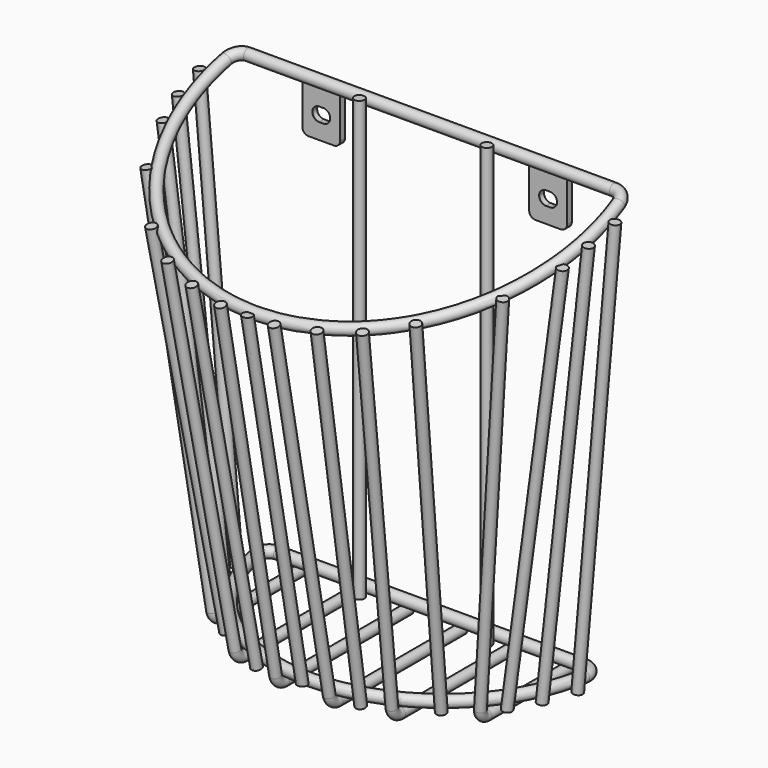
from build123d import *

# Parameters (mm, degrees)
F1_R           = 2.286
F3_R           = 2.0701
F4_DEPTH       = 177.1015
F4_DEPTH_BACK  = 2.286
F8_R           = 2.286
F15_R          = 2.0574
F23_R          = 2.0574
F31_R          = 2.0574
F38_R          = 2.0574
F47_R          = 2.0574
F48_DEPTH      = 154.305
F48_DEPTH_BACK = 1.27
F53_R          = 2.0574
F61_R          = 2.0574
F62_DEPTH      = 147.828
F62_DEPTH_BACK = 2.286
F65_R          = 2.0574
F68_R          = 2.0574
F71_W          = 15.4432
F71_H          = 22.0853
F72_DEPTH      = 2.032
F72_DEPTH_BACK = 0.4445
F73_R          = 2.54


with BuildPart() as f2:
    # F2: sweep along a path in F0
    with BuildLine(Plane.XY) as f2_path:
        Line((0, 0), (62.5051961959, 0))
        ThreePointArc((62.5051961959, 0), (65.9966185212, -1.6201947649), (67.0135070874, -5.3324715021))
        ThreePointArc((67.0135070874, -5.3324715021), (0, -61.9887), (-67.0135070874, -5.3324715021))
        ThreePointArc((-67.0135070874, -5.3324715021), (-65.9966185212, -1.6201947649), (-62.5051961959, 0))
        Line((-62.5051961959, 0), (0, 0))
    # F1 (on Right) → F2 (sweep)
    with BuildSketch(Plane.YZ):
        Circle(F1_R)
    sweep(path=f2_path.line)

    # F3 (on Top) → F4 (join, two sides)
    with BuildSketch(Plane.XY) as f4_sk:
        with Locations((-26.035, -4.064)):
            Circle(F3_R)
        with Locations((26.035, -4.064)):
            Circle(F3_R)
    extrude(amount=F4_DEPTH)
    extrude(f4_sk.sketch, amount=-F4_DEPTH_BACK)

    # F9: sweep along a path in F7
    with BuildLine(Plane(origin=(0, -55.5187618057, 155.4852954062), x_dir=(1, 0, 0), z_dir=(0, 0.3362735421, -0.9417643574))) as f9_path:
        Line((0, -58.1719834015), (74.751068181, -58.1719834015))
        ThreePointArc((74.751068181, -58.1719834015), (77.7736320182, -57.0303320499), (79.2866971284, -54.1755301423))
        ThreePointArc((79.2866971284, -54.1755301423), (0, 35.8080165985), (-79.2866971284, -54.1755301423))
        ThreePointArc((-79.2866971284, -54.1755301423), (-77.7736320182, -57.0303320499), (-74.751068181, -58.1719834015))
        Line((-74.751068181, -58.1719834015), (0, -58.1719834015))
    # F8 (on Right) → F9 (sweep)
    with BuildSketch(Plane.YZ):
        with Locations((0, 175.3235)):
            Circle(F8_R)
    sweep(path=f9_path.line)

    # F16: sweep along a path in F13
    with BuildLine(Plane(origin=(71.1091119248, 0, -6.2212411668), x_dir=(0, -1, 0), z_dir=(-0.9961946981, 0, 0.0871557427))) as f16_path:
        Line((12.2174, 3.9590052974), (12.2174, 178.5840052974))
    # F15 (on face) → F16 (sweep)
    with BuildSketch(Plane(origin=(0.5442880752, 0, 6.2212411668), x_dir=(0.9961946981, 0, -0.0871557427), z_dir=(0.0871557427, 0, 0.9961946981))):
        with Locations((69.596, -12.2174)):
            Circle(F15_R)
    sweep(path=f16_path.line)

    # F24: sweep along a path in F21
    with BuildLine(Plane(origin=(62.3644296008, -29.0810111193, -6.9289571848), x_dir=(-0.4179203376, -0.9072963082, 0.0464327525), z_dir=(-0.9017477159, 0.4204918657, 0.1001880616))) as f24_path:
        Line((0, 4.5939530634), (0, 176.0439530634))
    # F23 (on face) → F24 (sweep)
    with BuildSketch(Plane(origin=(0.6323393725, -0.294864692, 6.9289571848), x_dir=(0.9958690368, 0.0038605901, -0.090719113), z_dir=(0.0908012204, -0.0423413044, 0.9949685183))):
        with Locations((64.77, -24.3459)):
            Circle(F23_R)
    sweep(path=f24_path.line)

    # F32: sweep along a path in F29
    with BuildLine(Plane(origin=(56.1356379491, -39.3065968542, -7.6262052028), x_dir=(0.5648686384, 0.8216048417, -0.0767392036), z_dir=(0.8141263956, -0.5700574392, -0.1106016638))) as f32_path:
        Line((-2.934086835, 4.8319505917), (-2.934086835, 172.4719505917))
    # F31 (on face) → F32 (sweep)
    with BuildSketch(Plane(origin=(0.6951961369, -0.4867815756, 7.6262052028), x_dir=(0.9958874014, 0.0057712369, -0.0904155768), z_dir=(0.090599579, -0.0634385082, 0.9938648157))):
        with Locations((58.928, -34.8107)):
            Circle(F31_R)
    sweep(path=f32_path.line)

    # F39: sweep along a path in F36
    with BuildLine(Plane(origin=(53.621817871, 0, -6.1094344374), x_dir=(0, -1, 0), z_dir=(-0.9935718557, 0, 0.1132032138))) as f39_path:
        Line((-2.286, 1.2086064592), (39.3991410262, 1.2086064592))
        ThreePointArc((39.3991410262, 1.2086064592), (42.5172375284, 2.4368573354), (43.960003864, 5.4616798612))
        Line((43.960003864, 5.4616798612), (55.0908030935, 164.6395248132))
    # F38 (on offset) → F39 (sweep)
    with BuildSketch(Plane.XZ.offset(-2.286)):
        with Locations((54.3179, -4.191)):
            Circle(F38_R)
    sweep(path=f39_path.line)

    # F47 (on face) → F48 (join, two sides)
    with BuildSketch(Plane(origin=(0.6425642515, -1.6421882839, 9.8765288401), x_dir=(0.9979468925, 0.0105049647, -0.0631794711), z_dir=(0.0640468567, -0.1636832385, 0.984431713))) as f48_sk:
        with Locations((43.5737, -49.53)):
            Circle(F47_R)
    extrude(amount=F48_DEPTH)
    extrude(f48_sk.sketch, amount=-F48_DEPTH_BACK)

    # F54: sweep along a path in F52
    with BuildLine(Plane(origin=(31.9670002258, 0, -1.6753194922), x_dir=(0, -1, 0), z_dir=(-0.9986295348, 0, 0.0523359562))) as f54_path:
        Line((-2.3149095941, -2.5447886437), (55.5112067041, -2.5447886437))
        ThreePointArc((55.5112067041, -2.5447886437), (58.4652855391, -1.4622874956), (60.0205044744, 1.2726137023))
        Line((60.0205044744, 1.2726137023), (84.7445559985, 149.0177197445))
    # F53 (on offset) → F54 (sweep)
    with BuildSketch(Plane.XZ.offset(-2.286)):
        with Locations((31.877, -4.2926)):
            Circle(F53_R)
    sweep(path=f54_path.line)

    # F61 (on face) → F62 (join, two sides)
    with BuildSketch(Plane(origin=(0.3489269643, -2.2528747461, 11.9837463229), x_dir=(0.9995908303, 0.0052847552, -0.0281112678), z_dir=(-0.0286037063, 0.184682109, -0.9823819759))) as f62_sk:
        with Locations((21.0021745573, 61.8603080666)):
            Circle(F61_R)
    extrude(amount=-F62_DEPTH)
    extrude(f62_sk.sketch, amount=F62_DEPTH_BACK)

    # F66: sweep along a path in F64
    with BuildLine(Plane.YZ.offset(10.9601)) as f66_path:
        Line((2.286, -4.191), (-61.255134044, -4.191))
        ThreePointArc((-61.255134044, -4.191), (-64.1632836672, -3.1468675952), (-65.7431335268, -0.4913787269))
        Line((-65.7431335268, -0.4913787269), (-93.8609634713, 144.1623162344))
    # F65 (on offset) → F66 (sweep)
    with BuildSketch(Plane.XZ.offset(-2.286)):
        with Locations((10.9601, -4.191)):
            Circle(F65_R)
    sweep(path=f66_path.line)

    # F69: sweep along a path in F67
    with BuildLine(Plane.YZ) as f69_path:
        Line((-65.532, 0), (-93.5208174868, 143.989983404))
    # F68 (on Top) → F69 (sweep)
    with BuildSketch(Plane.XY):
        with Locations((0, -65.786)):
            Circle(F68_R)
    sweep(path=f69_path.line)

    # F70: F2 across plane


with BuildPart() as f2_1:
    add(f2.part)
    add(f2.part.mirror(Plane.YZ))

    # F71 (on offset) → F72 (join, two sides)
    with BuildSketch(Plane.XZ.offset(-2.286)) as f72_sk:
        with Locations((46.3296, 163.70935)):
            Rectangle(F71_W, F71_H)
        with BuildLine():
            ThreePointArc((47.18685, 164.7571), (49.1714866028, 163.9350366028), (49.99355, 161.9504))
            ThreePointArc((49.99355, 161.9504), (49.1714866028, 159.9657633972), (47.18685, 159.1437))
            Line((47.18685, 159.1437), (45.47235, 159.1437))
            ThreePointArc((45.47235, 159.1437), (43.4877133972, 159.9657633972), (42.66565, 161.9504))
            ThreePointArc((42.66565, 161.9504), (43.4877133972, 163.9350366028), (45.47235, 164.7571))
            Line((45.47235, 164.7571), (47.18685, 164.7571))
        make_face(mode=Mode.SUBTRACT)
        with Locations((-46.3296, 163.70935)):
            Rectangle(F71_W, F71_H)
        with BuildLine():
            Line((-47.18685, 164.7571), (-45.47235, 164.7571))
            ThreePointArc((-45.47235, 164.7571), (-43.4877133972, 163.9350366028), (-42.66565, 161.9504))
            ThreePointArc((-42.66565, 161.9504), (-43.4877133972, 159.9657633972), (-45.47235, 159.1437))
            Line((-45.47235, 159.1437), (-47.18685, 159.1437))
            ThreePointArc((-47.18685, 159.1437), (-49.1714866028, 159.9657633972), (-49.99355, 161.9504))
            ThreePointArc((-49.99355, 161.9504), (-49.1714866028, 163.9350366028), (-47.18685, 164.7571))
        make_face(mode=Mode.SUBTRACT)
    extrude(amount=-F72_DEPTH)
    extrude(f72_sk.sketch, amount=F72_DEPTH_BACK)

    # F73
    f73_edges = [f2_1.edges().sort_by_distance(p)[0] for p in [
        (-54.0512, 3.07975, 152.6667),
        (-38.608, 3.07975, 152.6667),
        (38.608, 3.07975, 152.6667),
        (54.0512, 3.07975, 152.6667),
    ]]
    fillet(f73_edges, radius=F73_R)


solid = f2_1.part
